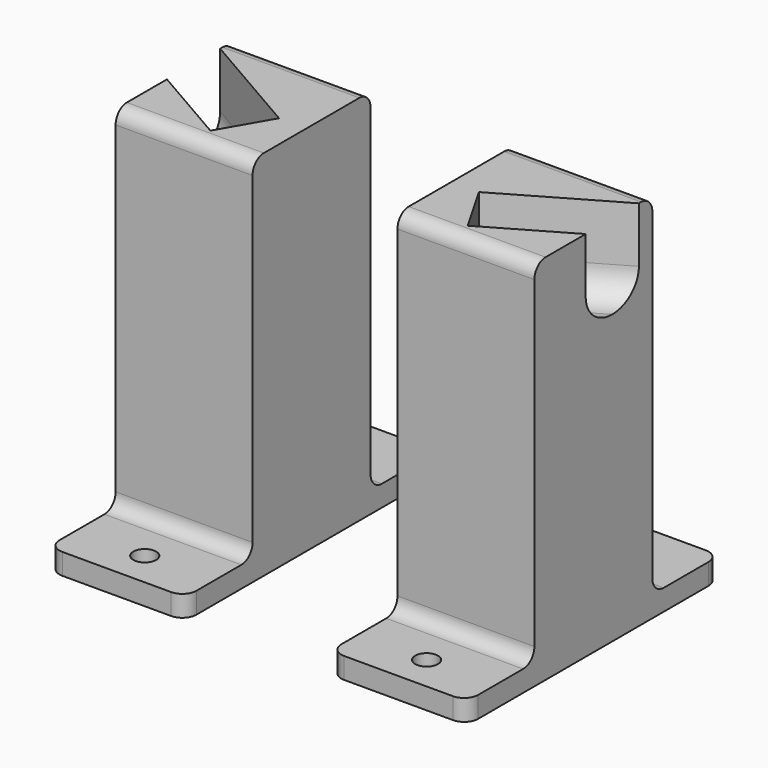
from build123d import *

# Parameters (mm, degrees)
F0_W     = 19.5
F0_H     = 45
F1_DEPTH = 3
F2_D     = 3.25
F3_D     = 3.25
F4_W     = 19.5
F4_H     = 21
F5_DEPTH = 50
F6_R     = 2
F7_R     = 2
F9_DEPTH = 12
F10_R    = 4.09999
F11_R    = 2


# Not quite as in the source:
# - a fillet or chamfer is up to 0.001 mm smaller than in the source, because OpenCascade refuses the exact size


with BuildPart() as f1:
    # F0 (on Top) → F1 (new body)
    with BuildSketch(Plane.XY):
        with Locations((-20.0667725876, 1.1574134253)):
            Rectangle(F0_W, F0_H)
    extrude(amount=F1_DEPTH)

    # F2 (through all)
    with Locations(Plane(origin=(0, 0, 0), x_dir=(1, 0, 0), z_dir=(0, 0, -1))):
        with Locations((-20.0667725876, 16.3425865747)):
            Hole(F2_D / 2)

    # F3 (through all)
    with Locations(Plane(origin=(0, 0, 0), x_dir=(1, 0, 0), z_dir=(0, 0, -1))):
        with Locations((-20.0667725876, -18.6574134253)):
            Hole(F3_D / 2)

    # F4 (on face) → F5 (join)
    with BuildSketch(Plane.XY.offset(3)):
        with Locations((-20.0667725876, 1.1574134253)):
            Rectangle(F4_W, F4_H)
    extrude(amount=F5_DEPTH)

    # F6
    f6_edges = [f1.edges().sort_by_distance(p)[0] for p in [
        (-20.066773, -9.342587, 3),
        (-20.066773, 11.657413, 3),
    ]]
    fillet(f6_edges, radius=F6_R)

    # F7
    f7_edges = [f1.edges().sort_by_distance(p)[0] for p in [
        (-10.316773, -21.342587, 1.5),
        (-29.816773, -21.342587, 1.5),
        (-10.316773, 23.657413, 1.5),
        (-29.816773, 23.657413, 1.5),
    ]]
    fillet(f7_edges, radius=F7_R)

    # F8 (on face) → F9 (cut)
    with BuildSketch(Plane.XY.offset(53)):
        Polygon((-14.2283153195, 0.2588217364), (-29.8167725876, 9.2588217364), (-29.8167725876, -0.2097226783), (-18.3283153195, -6.8425865747), align=None)
    extrude(amount=-F9_DEPTH, mode=Mode.SUBTRACT)

    # F10 (radius 4.1 in the source; OpenCascade refuses exactly that, so slightly less here)
    f10_edges = [f1.edges().sort_by_distance(p)[0] for p in [
        (-22.022544, 4.758822, 41),
        (-24.072544, -3.526155, 41),
    ]]
    fillet(f10_edges, radius=F10_R)

    # F11
    f11_edges = [f1.edges().sort_by_distance(p)[0] for p in [
        (-20.066773, -9.342587, 53),
        (-20.066773, 11.657413, 53),
    ]]
    fillet(f11_edges, radius=F11_R)


with BuildPart() as f12_1:
    # F12: instance of F1
    add(f1.part.mirror(Plane.YZ))


solid = Compound([f1.part, f12_1.part])
